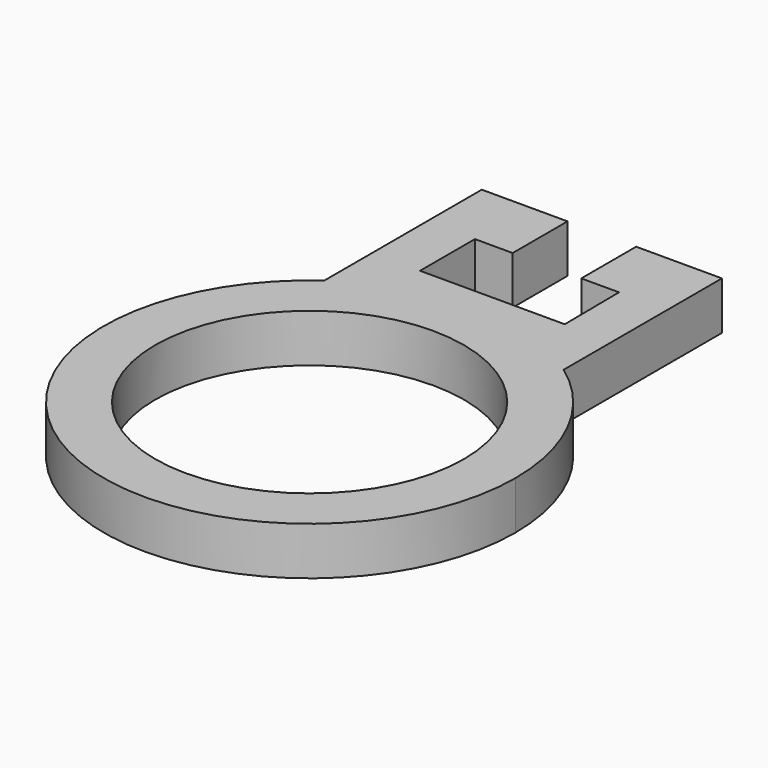
from build123d import *

# Parameters (mm, degrees)
F0_R     = 45
F1_DEPTH = 14


with BuildPart() as f1:
    # F0 (on Top) → F1 (new body)
    with BuildSketch(Plane.XY):
        with BuildLine():
            ThreePointArc((-34.8038087036, 48.8742764624), (-27.493376273, -53.3302377747), (60, 0))
            ThreePointArc((60, 0), (53.4404878242, 27.2784578213), (35.1961912964, 48.5924697688))
            Line((35.1961912964, 48.5924697688), (-34.8038087036, 48.5924697688))
            Line((-34.8038087036, 48.5924697688), (-34.8038087036, 48.8742764624))
        make_face()
        Circle(F0_R, mode=Mode.SUBTRACT)
        with BuildLine():
            Line((-34.8038087036, 48.5924697688), (35.1961912964, 48.5924697688))
            ThreePointArc((35.1961912964, 48.5924697688), (0.2415466371, 59.9995137915), (-34.8038087036, 48.8742764624))
            Line((-34.8038087036, 48.8742764624), (-34.8038087036, 48.5924697688))
        make_face()
        with BuildLine():
            ThreePointArc((-34.8038087036, 48.8742764624), (0.2415466371, 59.9995137915), (35.1961912964, 48.5924697688))
            Line((35.1961912964, 48.5924697688), (35.1961912964, 66.2418827415))
            Line((35.1961912964, 66.2418827415), (21.3984008878, 66.2418827415))
            Line((21.3984008878, 66.2418827415), (-20.8038087036, 66.2418827415))
            Line((-20.8038087036, 66.2418827415), (-34.8038087036, 66.2418827415))
            Line((-34.8038087036, 66.2418827415), (-34.8038087036, 48.8742764624))
        make_face()
        Polygon((21.3984008878, 66.2418827415), (35.1961912964, 66.2418827415), (35.1961912964, 106.2418827415), (10.1961912964, 106.2418827415), (10.1961912964, 86.2418827415), (21.1961912964, 86.2418827415), align=None)
        Polygon((-34.8038087036, 106.2418827415), (-34.8038087036, 66.2418827415), (-20.8038087036, 66.2418827415), (-20.8038087036, 86.2418827415), (-9.8038087036, 86.2418827415), (-9.8038087036, 106.2418827415), align=None)
    extrude(amount=F1_DEPTH)


solid = f1.part
